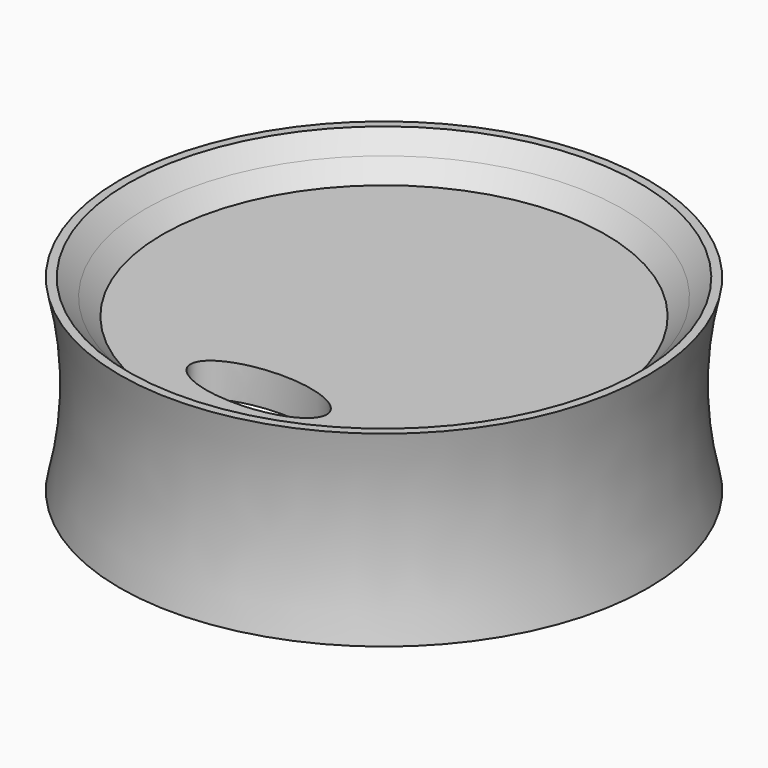
from build123d import *

# Parameters (mm, degrees)
F3_DEPTH = 65.786
F4_SIZE  = 2.53999


# Not quite as in the source:
# - a fillet or chamfer is up to 0.001 mm smaller than in the source, because OpenCascade refuses the exact size


with BuildPart() as f1:
    # F0 (on Front) → F1 (revolve)
    with BuildSketch(Plane.XZ):
        with BuildLine():
            Line((-39.4843606797, -37.7460680902), (-31.8643606797, -37.7460680902))
            Line((-31.8643606797, -37.7460680902), (-31.8643606797, -19.9660680902))
            Line((-31.8643606797, -19.9660680902), (-0.1143606797, -19.9660680902))
            Line((-0.1143606797, -19.9660680902), (-0.1143606797, -14.8860680902))
            Line((-0.1143606797, -14.8860680902), (-35.6743606797, -14.8860680902))
            Line((-35.6743606797, -14.8860680902), (-35.6743606797, -9.8060680902))
            Line((-35.6743606797, -9.8060680902), (-39.4843606797, -9.8060680902))
            ThreePointArc((-39.4843606797, -9.8060680902), (-37.8052347612, -23.7760680902), (-39.4843606797, -37.7460680902))
        make_face()
    revolve(axis=Axis((-0.1143606797, 0, -17.4260680902), (0, 0, -1)))

    # F2 (on Top) → F3 (cut)
    with BuildSketch(Plane.XY):
        with BuildLine():
            add(Edge.make_bspline(
                [(10.16, -23.495), (10.16, -15.7960341604), (-5.08, -19.6455170802), (-20.32, -23.495), (-5.08, -27.3444829198), (10.16, -31.1939658396), (10.16, -23.495)],
                knots=[0, 0, 0, 2.0943951024, 2.0943951024, 4.1887902048, 4.1887902048, 6.2831853072, 6.2831853072, 6.2831853072], degree=2, weights=[1, 0.5, 1, 0.5, 1, 0.5, 1]))
        make_face()
    extrude(amount=-F3_DEPTH, mode=Mode.SUBTRACT)

    # F4 (size 2.54 in the source; OpenCascade refuses exactly that, so slightly less here)
    f4_edges = [f1.edges().sort_by_distance(p)[0] for p in [
        (35.445639, 0, -14.886068),
        (35.445639, 0, -9.806068),
        (-35.674361, 0, -12.346068),
    ]]
    chamfer(f4_edges, length=F4_SIZE)


solid = f1.part
